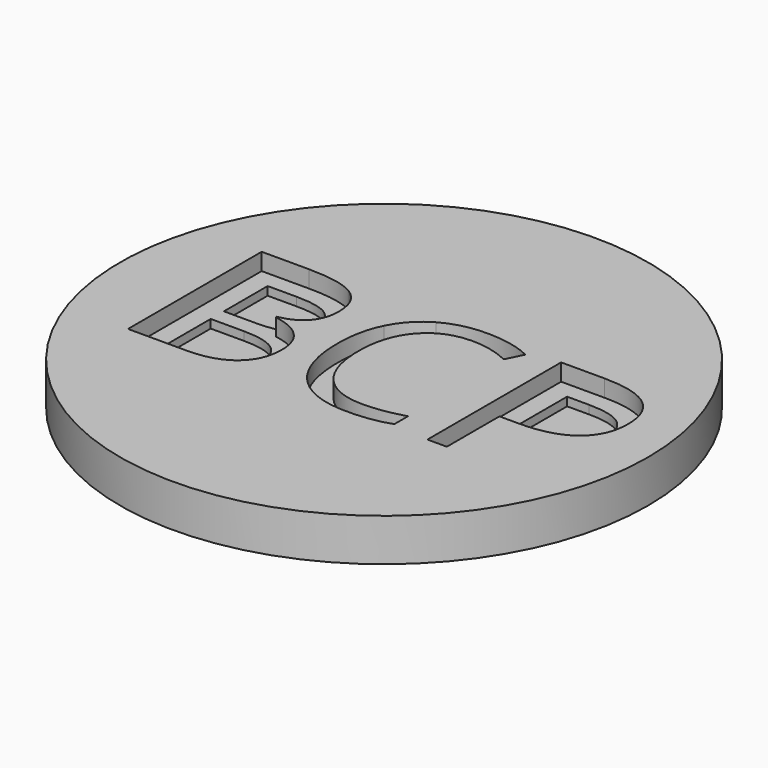
from build123d import *

# Parameters (mm, degrees)
F0_R         = 7.874
F1_DEPTH     = 1.27
F0_TEXT_SIZE = 6.9843889731
F2_DEPTH     = 0.762
F3_DEPTH     = 0.508


# Not quite as in the source:
# - Text() gives the source's letters only with a copy of the font that has no kerning and outlines rounded to 1/6400 em; it was checked with that copy


with BuildPart() as f1:
    # F0 (on Top) → F1 (new body)
    with BuildSketch(Plane.XY):
        Circle(F0_R)
        with BuildLine():
            Line((-5.6305101041, -2.5116563775), (-5.6305101041, 2.4745425629))
            Line((-5.6305101041, 2.4745425629), (-4.2216278909, 2.4745425629))
            add(Edge.make_bspline(
                [(-4.2216278909, 2.4745425629), (-3.2296263946, 2.4745425629), (-2.7860085637, 2.1777060315)],
                knots=[0, 0, 0, 1, 1, 1], degree=2))
            add(Edge.make_bspline(
                [(-2.7860085637, 2.1777060315), (-2.3423907328, 1.8808695002), (-2.3423907328, 1.240270074)],
                knots=[0, 0, 0, 1, 1, 1], degree=2))
            add(Edge.make_bspline(
                [(-2.3423907328, 1.240270074), (-2.3423907328, 0.7961065878), (-2.5895726238, 0.5080005426)],
                knots=[0, 0, 0, 1, 1, 1], degree=2))
            add(Edge.make_bspline(
                [(-2.5895726238, 0.5080005426), (-2.8367545148, 0.2198944975), (-3.3114747029, 0.1347722569)],
                knots=[0, 0, 0, 1, 1, 1], degree=2))
            Line((-3.3114747029, 0.1347722569), (-3.3114747029, 0.1009416228))
            add(Edge.make_bspline(
                [(-3.3114747029, 0.1009416228), (-2.175420184, -0.0933116955), (-2.175420184, -1.0929523673)],
                knots=[0, 0, 0, 1, 1, 1], degree=2))
            add(Edge.make_bspline(
                [(-2.175420184, -1.0929523673), (-2.175420184, -1.7608345629), (-2.6272228457, -2.1362454702)],
                knots=[0, 0, 0, 1, 1, 1], degree=2))
            add(Edge.make_bspline(
                [(-2.6272228457, -2.1362454702), (-3.0790255074, -2.5116563775), (-3.8909607255, -2.5116563775)],
                knots=[0, 0, 0, 1, 1, 1], degree=2))
            Line((-3.8909607255, -2.5116563775), (-5.6305101041, -2.5116563775))
        make_face(mode=Mode.SUBTRACT)
        with BuildLine():
            add(Edge.make_bspline(
                [(2.1625401548, 1.7619166255), (1.5961498615, 2.0271051443), (1.0297595683, 2.0271051443)],
                knots=[0, 0, 0, 1, 1, 1], degree=2))
            add(Edge.make_bspline(
                [(1.0297595683, 2.0271051443), (0.2080025531, 2.0271051443), (-0.2678089457, 1.4798127896)],
                knots=[0, 0, 0, 1, 1, 1], degree=2))
            add(Edge.make_bspline(
                [(-0.2678089457, 1.4798127896), (-0.7436204445, 0.9325204349), (-0.7436204445, -0.0191025627)],
                knots=[0, 0, 0, 1, 1, 1], degree=2))
            add(Edge.make_bspline(
                [(-0.7436204445, -0.0191025627), (-0.7436204445, -0.9969170189), (-0.2847242627, -1.5311136443)],
                knots=[0, 0, 0, 1, 1, 1], degree=2))
            add(Edge.make_bspline(
                [(-0.2847242627, -1.5311136443), (0.174171919, -2.0653102696), (1.0232117036, -2.0653102696)],
                knots=[0, 0, 0, 1, 1, 1], degree=2))
            add(Edge.make_bspline(
                [(1.0232117036, -2.0653102696), (1.544858255, -2.0653102696), (2.2138317614, -1.877604816)],
                knots=[0, 0, 0, 1, 1, 1], degree=2))
            Line((2.2138317614, -1.877604816), (2.2138317614, -2.3850643273))
            add(Edge.make_bspline(
                [(2.2138317614, -2.3850643273), (1.6954591423, -2.5804089564), (0.9348155307, -2.5804089564)],
                knots=[0, 0, 0, 1, 1, 1], degree=2))
            add(Edge.make_bspline(
                [(0.9348155307, -2.5804089564), (-0.1663170434, -2.5804089564), (-0.7649010046, -1.9114354501)],
                knots=[0, 0, 0, 1, 1, 1], degree=2))
            add(Edge.make_bspline(
                [(-0.7649010046, -1.9114354501), (-1.3634849658, -1.2424619437), (-1.3634849658, -0.0114633872)],
                knots=[0, 0, 0, 1, 1, 1], degree=2))
            add(Edge.make_bspline(
                [(-1.3634849658, -0.0114633872), (-1.3634849658, 0.7590020214), (-1.0753789207, 1.338488044)],
                knots=[0, 0, 0, 1, 1, 1], degree=2))
            add(Edge.make_bspline(
                [(-1.0753789207, 1.338488044), (-0.7872728755, 1.9179740666), (-0.2432544532, 2.231725915)],
                knots=[0, 0, 0, 1, 1, 1], degree=2))
            add(Edge.make_bspline(
                [(-0.2432544532, 2.231725915), (0.3007639692, 2.5454777634), (1.0373987437, 2.5454777634)],
                knots=[0, 0, 0, 1, 1, 1], degree=2))
            add(Edge.make_bspline(
                [(1.0373987437, 2.5454777634), (1.8209598816, 2.5454777634), (2.4080850797, 2.2595543398)],
                knots=[0, 0, 0, 1, 1, 1], degree=2))
            Line((2.4080850797, 2.2595543398), (2.1625401548, 1.7619166255))
        make_face(mode=Mode.SUBTRACT)
        with BuildLine():
            add(Edge.make_bspline(
                [(4.5950718769, 2.4745425629), (6.4633959272, 2.4745425629), (6.4633959272, 1.0220079186)],
                knots=[0, 0, 0, 1, 1, 1], degree=2))
            add(Edge.make_bspline(
                [(6.4633959272, 1.0220079186), (6.4633959272, 0.2646382394), (5.9466602743, -0.1429663359)],
                knots=[0, 0, 0, 1, 1, 1], degree=2))
            add(Edge.make_bspline(
                [(5.9466602743, -0.1429663359), (5.4299246213, -0.5505709111), (4.4684798268, -0.5505709111)],
                knots=[0, 0, 0, 1, 1, 1], degree=2))
            Line((4.4684798268, -0.5505709111), (3.8813546287, -0.5505709111))
            Line((3.8813546287, -0.5505709111), (3.8813546287, -2.5116563775))
            Line((3.8813546287, -2.5116563775), (3.3018686061, -2.5116563775))
            Line((3.3018686061, -2.5116563775), (3.3018686061, 2.4745425629))
            Line((3.3018686061, 2.4745425629), (4.5950718769, 2.4745425629))
        make_face(mode=Mode.SUBTRACT)
    extrude(amount=F1_DEPTH)

    # F0 (on Top) → F2 (join)
    with BuildSketch(Plane.XY):
        with Locations((-6.3158532721, -2.5116563775)):
            Text('BCP', F0_TEXT_SIZE, font='Open Sans', text_align=(TextAlign.LEFT, TextAlign.BOTTOM))
    extrude(amount=F2_DEPTH)

    # F0 (on Top) → F3 (join)
    with BuildSketch(Plane.XY):
        with BuildLine():
            Line((-4.0579312744, -0.1511511667), (-5.0510240815, -0.1511511667))
            Line((-5.0510240815, -0.1511511667), (-5.0510240815, -2.0172925955))
            Line((-5.0510240815, -2.0172925955), (-4.0099136002, -2.0172925955))
            add(Edge.make_bspline(
                [(-4.0099136002, -2.0172925955), (-3.4064187405, -2.0172925955), (-3.1013973783, -1.7837520892)],
                knots=[0, 0, 0, 1, 1, 1], degree=2))
            add(Edge.make_bspline(
                [(-3.1013973783, -1.7837520892), (-2.7963760161, -1.5502115829), (-2.7963760161, -1.0514825578)],
                knots=[0, 0, 0, 1, 1, 1], degree=2))
            add(Edge.make_bspline(
                [(-2.7963760161, -1.0514825578), (-2.7963760161, -0.5876754775), (-3.1084908983, -0.3694133221)],
                knots=[0, 0, 0, 1, 1, 1], degree=2))
            add(Edge.make_bspline(
                [(-3.1084908983, -0.3694133221), (-3.4206057806, -0.1511511667), (-4.0579312744, -0.1511511667)],
                knots=[0, 0, 0, 1, 1, 1], degree=2))
        make_face()
        with BuildLine():
            Line((-5.0510240815, 1.9725396055), (-5.0510240815, 0.339938683))
            Line((-5.0510240815, 0.339938683), (-4.0961271516, 0.339938683))
            add(Edge.make_bspline(
                [(-4.0961271516, 0.339938683), (-3.4817191841, 0.339938683), (-3.2121654222, 0.5325550351)],
                knots=[0, 0, 0, 1, 1, 1], degree=2))
            add(Edge.make_bspline(
                [(-3.2121654222, 0.5325550351), (-2.9426116602, 0.7251713873), (-2.9426116602, 1.1813392921)],
                knots=[0, 0, 0, 1, 1, 1], degree=2))
            add(Edge.make_bspline(
                [(-2.9426116602, 1.1813392921), (-2.9426116602, 1.6014939413), (-3.2427221239, 1.7870167734)],
                knots=[0, 0, 0, 1, 1, 1], degree=2))
            add(Edge.make_bspline(
                [(-3.2427221239, 1.7870167734), (-3.5428325876, 1.9725396055), (-4.1976190538, 1.9725396055)],
                knots=[0, 0, 0, 1, 1, 1], degree=2))
            Line((-4.1976190538, 1.9725396055), (-5.0510240815, 1.9725396055))
        make_face()
        with BuildLine():
            Line((3.8813546287, 1.9725396055), (3.8813546287, -0.0529331968))
            Line((3.8813546287, -0.0529331968), (4.4040924909, -0.0529331968))
            add(Edge.make_bspline(
                [(4.4040924909, -0.0529331968), (5.1745578995, -0.0529331968), (5.5188664497, 0.1958856604)],
                knots=[0, 0, 0, 1, 1, 1], degree=2))
            add(Edge.make_bspline(
                [(5.5188664497, 0.1958856604), (5.8631749998, 0.4447045176), (5.8631749998, 0.9947251492)],
                knots=[0, 0, 0, 1, 1, 1], degree=2))
            add(Edge.make_bspline(
                [(5.8631749998, 0.9947251492), (5.8631749998, 1.4890889312), (5.539055699, 1.7308142683)],
                knots=[0, 0, 0, 1, 1, 1], degree=2))
            add(Edge.make_bspline(
                [(5.539055699, 1.7308142683), (5.2149363983, 1.9725396055), (4.5295932303, 1.9725396055)],
                knots=[0, 0, 0, 1, 1, 1], degree=2))
            Line((4.5295932303, 1.9725396055), (3.8813546287, 1.9725396055))
        make_face()
    extrude(amount=F3_DEPTH)


solid = f1.part
